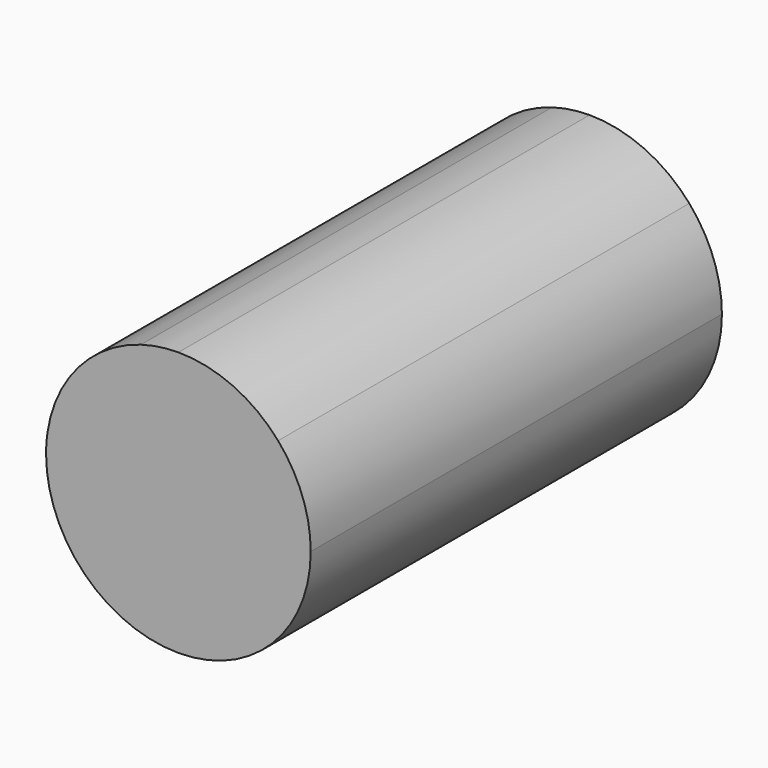
from build123d import *

# Parameters (mm, degrees)
F1_DEPTH = 37


with BuildPart() as f1:
    # F0 (on Front) → F1 (new body, symmetric)
    with BuildSketch(Plane.XZ):
        with BuildLine():
            ThreePointArc((-137.570944, -62.912574), (-118.520944, -81.962574), (-99.470944, -62.912574))
            Line((-99.470944, -62.912574), (-118.520944, -62.912574))
            Line((-118.520944, -62.912574), (-137.570944, -62.912574))
        make_face()
        with BuildLine():
            ThreePointArc((-99.470944, -62.912574), (-100.683018, -56.225954), (-104.165001, -50.390218))
            ThreePointArc((-104.165001, -50.390218), (-110.635781, -45.571101), (-118.520944, -43.862574))
            Line((-118.520944, -43.862574), (-118.520944, -62.912574))
            Line((-118.520944, -62.912574), (-99.470944, -62.912574))
        make_face()
        with BuildLine():
            Line((-137.375208, -60.188746), (-118.520944, -62.912574))
            Line((-118.520944, -62.912574), (-123.931437, -44.647058))
            ThreePointArc((-123.931437, -44.647058), (-132.928602, -50.449754), (-137.375208, -60.188746))
        make_face()
        with BuildLine():
            Line((-118.520944, -62.912574), (-118.520944, -43.862574))
            ThreePointArc((-118.520944, -43.862574), (-121.254479, -44.059715), (-123.931437, -44.647058))
            Line((-123.931437, -44.647058), (-118.520944, -62.912574))
        make_face()
        with BuildLine():
            Line((-137.570944, -62.912574), (-118.520944, -62.912574))
            Line((-118.520944, -62.912574), (-137.375208, -60.188746))
            ThreePointArc((-137.375208, -60.188746), (-137.521947, -61.547148), (-137.570944, -62.912574))
        make_face()
    extrude(amount=F1_DEPTH, both=True)


solid = f1.part
